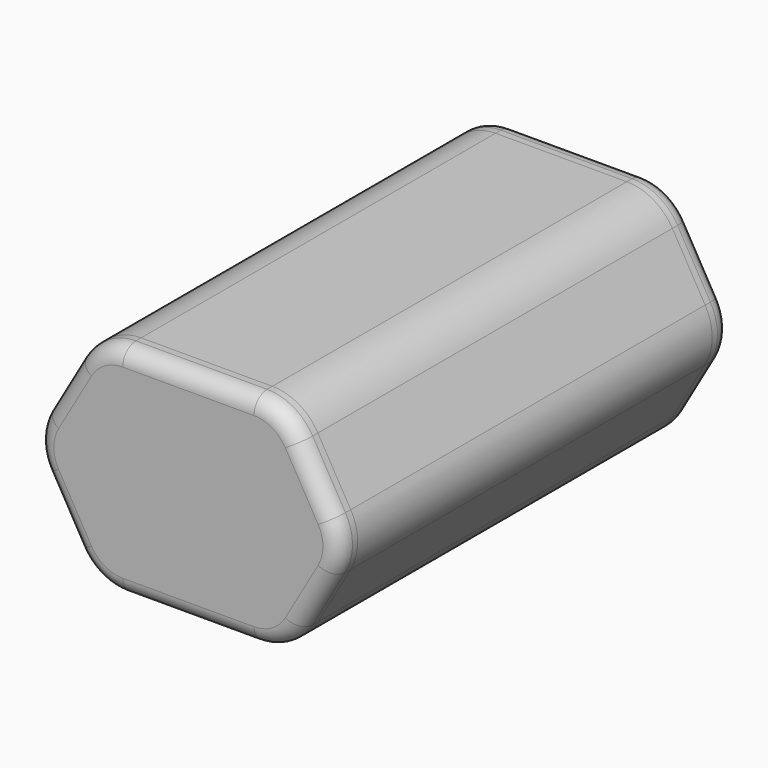
from build123d import *

# Parameters (mm, degrees)
F0_R      = 9
F4_DEPTH  = 65
F3_R      = 9
F5_DEPTH  = 65
F6_DEPTH  = 135
F8_DEPTH  = 5
F10_DEPTH = 2
F11_R     = 5
F12_R     = 4.99999


# Not quite as in the source:
# - a fillet or chamfer is up to 0.001 mm smaller than in the source, because OpenCascade refuses the exact size


with BuildPart() as f4:
    # F0 (on Front) → F4 (new body)
    with BuildSketch(Plane.XZ):
        Circle(F0_R)
    extrude(amount=-F4_DEPTH)


with BuildPart() as f5:
    # F3 (on offset) → F5 (new body)
    with BuildSketch(Plane.XZ.offset(-70)):
        Circle(F3_R)
    extrude(amount=-F5_DEPTH)


with BuildPart() as f6:
    # F1 (on Front) → F6 (new body)
    with BuildSketch(Plane.XZ):
        with BuildLine():
            Line((50, 33.3205080757), (10, 33.3205080757))
            ThreePointArc((10, 33.3205080757), (2, 31.1769145362), (-3.8564064606, 25.3205080757))
            Line((-3.8564064606, 25.3205080757), (-13.8564064606, 8))
            ThreePointArc((-13.8564064606, 8), (-16, 0), (-13.8564064606, -8))
            Line((-13.8564064606, -8), (-3.8564064606, -25.3205080757))
            ThreePointArc((-3.8564064606, -25.3205080757), (2, -31.1769145362), (10, -33.3205080757))
            Line((10, -33.3205080757), (50, -33.3205080757))
            ThreePointArc((50, -33.3205080757), (58, -31.1769145362), (63.8564064606, -25.3205080757))
            Line((63.8564064606, -25.3205080757), (73.8564064606, -8))
            ThreePointArc((73.8564064606, -8), (76, 0), (73.8564064606, 8))
            Line((73.8564064606, 8), (63.8564064606, 25.3205080757))
            ThreePointArc((63.8564064606, 25.3205080757), (58, 31.1769145362), (50, 33.3205080757))
        make_face()
        with BuildLine():
            ThreePointArc((-2.124355653, 24.3205080757), (3, 29.4448637287), (10, 31.3205080757))
            Line((10, 31.3205080757), (50, 31.3205080757))
            ThreePointArc((50, 31.3205080757), (57, 29.4448637287), (62.124355653, 24.3205080757))
            Line((62.124355653, 24.3205080757), (72.124355653, 7))
            ThreePointArc((72.124355653, 7), (74, 0), (72.124355653, -7))
            Line((72.124355653, -7), (62.124355653, -24.3205080757))
            ThreePointArc((62.124355653, -24.3205080757), (57, -29.4448637287), (50, -31.3205080757))
            Line((50, -31.3205080757), (10, -31.3205080757))
            ThreePointArc((10, -31.3205080757), (3, -29.4448637287), (-2.124355653, -24.3205080757))
            Line((-2.124355653, -24.3205080757), (-12.124355653, -7))
            ThreePointArc((-12.124355653, -7), (-14, 0), (-12.124355653, 7))
            Line((-12.124355653, 7), (-2.124355653, 24.3205080757))
        make_face(mode=Mode.SUBTRACT)
    extrude(amount=-F6_DEPTH)


with BuildPart() as f8:
    # F7 (on face) → F8 (new body)
    with BuildSketch(Plane.XZ):
        with BuildLine():
            ThreePointArc((-3.8564064606, -25.3205080757), (2, -31.1769145362), (10, -33.3205080757))
            Line((10, -33.3205080757), (50, -33.3205080757))
            ThreePointArc((50, -33.3205080757), (58, -31.1769145362), (63.8564064606, -25.3205080757))
            Line((63.8564064606, -25.3205080757), (73.8564064606, -8))
            ThreePointArc((73.8564064606, -8), (76, 0), (73.8564064606, 8))
            Line((73.8564064606, 8), (63.8564064606, 25.3205080757))
            ThreePointArc((63.8564064606, 25.3205080757), (58, 31.1769145362), (50, 33.3205080757))
            Line((50, 33.3205080757), (10, 33.3205080757))
            ThreePointArc((10, 33.3205080757), (2, 31.1769145362), (-3.8564064606, 25.3205080757))
            Line((-3.8564064606, 25.3205080757), (-13.8564064606, 8))
            ThreePointArc((-13.8564064606, 8), (-16, 0), (-13.8564064606, -8))
            Line((-13.8564064606, -8), (-3.8564064606, -25.3205080757))
        make_face()
        with BuildLine():
            ThreePointArc((-2.124355653, 24.3205080757), (3, 29.4448637287), (10, 31.3205080757))
            Line((10, 31.3205080757), (50, 31.3205080757))
            ThreePointArc((50, 31.3205080757), (57, 29.4448637287), (62.124355653, 24.3205080757))
            Line((62.124355653, 24.3205080757), (72.124355653, 7))
            ThreePointArc((72.124355653, 7), (74, 0), (72.124355653, -7))
            Line((72.124355653, -7), (62.124355653, -24.3205080757))
            ThreePointArc((62.124355653, -24.3205080757), (57, -29.4448637287), (50, -31.3205080757))
            Line((50, -31.3205080757), (10, -31.3205080757))
            ThreePointArc((10, -31.3205080757), (3, -29.4448637287), (-2.124355653, -24.3205080757))
            Line((-2.124355653, -24.3205080757), (-12.124355653, -7))
            ThreePointArc((-12.124355653, -7), (-14, 0), (-12.124355653, 7))
            Line((-12.124355653, 7), (-2.124355653, 24.3205080757))
        make_face(mode=Mode.SUBTRACT)
    extrude(amount=F8_DEPTH)

    # F9 (on face) → F10 (join)
    with BuildSketch(Plane.XZ.offset(5)):
        with BuildLine():
            Line((-13.8564064606, -8), (-3.8564064606, -25.3205080757))
            ThreePointArc((-3.8564064606, -25.3205080757), (2, -31.1769145362), (10, -33.3205080757))
            Line((10, -33.3205080757), (50, -33.3205080757))
            ThreePointArc((50, -33.3205080757), (58, -31.1769145362), (63.8564064606, -25.3205080757))
            Line((63.8564064606, -25.3205080757), (73.8564064606, -8))
            ThreePointArc((73.8564064606, -8), (76, 0), (73.8564064606, 8))
            Line((73.8564064606, 8), (63.8564064606, 25.3205080757))
            ThreePointArc((63.8564064606, 25.3205080757), (58, 31.1769145362), (50, 33.3205080757))
            Line((50, 33.3205080757), (10, 33.3205080757))
            ThreePointArc((10, 33.3205080757), (2, 31.1769145362), (-3.8564064606, 25.3205080757))
            Line((-3.8564064606, 25.3205080757), (-13.8564064606, 8))
            ThreePointArc((-13.8564064606, 8), (-16, 0), (-13.8564064606, -8))
        make_face()
        with BuildLine():
            Line((-12.124355653, 7), (-2.124355653, 24.3205080757))
            ThreePointArc((-2.124355653, 24.3205080757), (3, 29.4448637287), (10, 31.3205080757))
            Line((10, 31.3205080757), (50, 31.3205080757))
            ThreePointArc((50, 31.3205080757), (57, 29.4448637287), (62.124355653, 24.3205080757))
            Line((62.124355653, 24.3205080757), (72.124355653, 7))
            ThreePointArc((72.124355653, 7), (74, 0), (72.124355653, -7))
            Line((72.124355653, -7), (62.124355653, -24.3205080757))
            ThreePointArc((62.124355653, -24.3205080757), (57, -29.4448637287), (50, -31.3205080757))
            Line((50, -31.3205080757), (10, -31.3205080757))
            ThreePointArc((10, -31.3205080757), (3, -29.4448637287), (-2.124355653, -24.3205080757))
            Line((-2.124355653, -24.3205080757), (-12.124355653, -7))
            ThreePointArc((-12.124355653, -7), (-14, 0), (-12.124355653, 7))
        make_face(mode=Mode.SUBTRACT)
        with BuildLine():
            ThreePointArc((10, 31.3205080757), (3, 29.4448637287), (-2.124355653, 24.3205080757))
            Line((-2.124355653, 24.3205080757), (-12.124355653, 7))
            ThreePointArc((-12.124355653, 7), (-14, 0), (-12.124355653, -7))
            Line((-12.124355653, -7), (-2.124355653, -24.3205080757))
            ThreePointArc((-2.124355653, -24.3205080757), (3, -29.4448637287), (10, -31.3205080757))
            Line((10, -31.3205080757), (50, -31.3205080757))
            ThreePointArc((50, -31.3205080757), (57, -29.4448637287), (62.124355653, -24.3205080757))
            Line((62.124355653, -24.3205080757), (72.124355653, -7))
            ThreePointArc((72.124355653, -7), (74, 0), (72.124355653, 7))
            Line((72.124355653, 7), (62.124355653, 24.3205080757))
            ThreePointArc((62.124355653, 24.3205080757), (57, 29.4448637287), (50, 31.3205080757))
            Line((50, 31.3205080757), (10, 31.3205080757))
        make_face()
    extrude(amount=F10_DEPTH)

    # F11
    f11_edges = [f8.edges().sort_by_distance(p)[0] for p in [
        (2, -7, 31.176915),
        (-8.856406, -7, 16.660254),
        (-16, -7, 0),
        (-8.856406, -7, -16.660254),
        (2, -7, -31.176915),
        (30, -7, -33.320508),
        (58, -7, -31.176915),
        (68.856406, -7, -16.660254),
        (76, -7, 0),
        (68.856406, -7, 16.660254),
        (58, -7, 31.176915),
        (30, -7, 33.320508),
    ]]
    fillet(f11_edges, radius=F11_R)

    # F12 (radius 5 in the source; OpenCascade refuses exactly that, so slightly less here)
    f12_edges = [f8.edges().sort_by_distance(p)[0] for p in [
        (3, -5, 29.444864),
        (30, -5, 31.320508),
        (57, -5, 29.444864),
        (67.124356, -5, 15.660254),
        (74, -5, 0),
        (67.124356, -5, -15.660254),
        (57, -5, -29.444864),
        (30, -5, -31.320508),
        (3, -5, -29.444864),
        (-7.124356, -5, -15.660254),
        (-14, -5, 0),
        (-7.124356, -5, 15.660254),
    ]]
    fillet(f12_edges, radius=F12_R)


with BuildPart() as f14_1:
    # F14: instance of F8
    add(f8.part.mirror(Plane.XZ.offset(-67.5)))


solid = Compound([f4.part, f5.part, f6.part, f8.part, f14_1.part])
